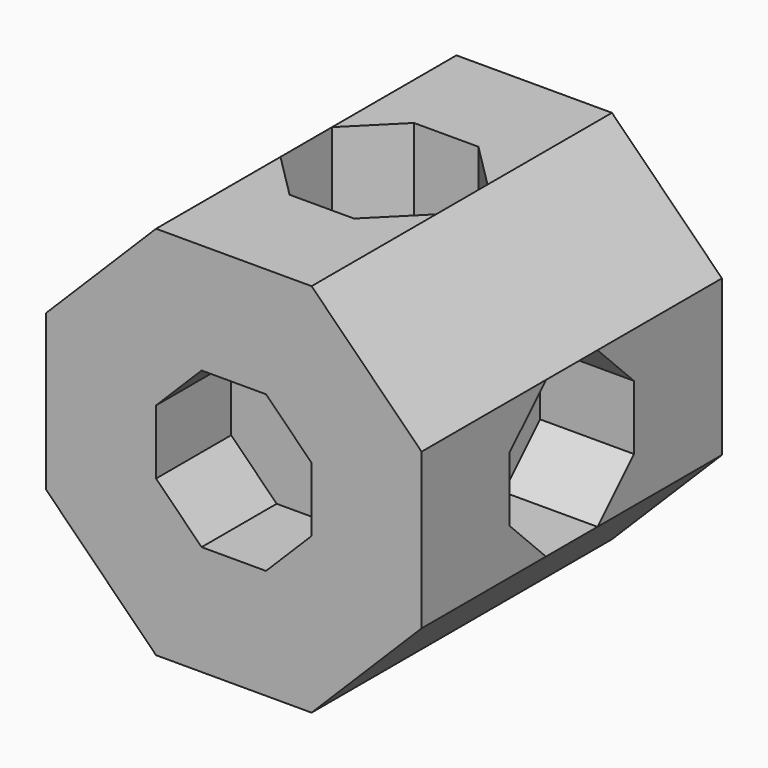
from build123d import *

# Parameters (mm, degrees)
F1_DEPTH        = 15
F2_DEPTH        = 20
F3_DEPTH        = 5
F5_DEPTH        = 5
F5_COPIES_COUNT = 4


# Not quite as in the source:
# - a pattern or mirror of a feature is missing from the dataset's text; its kind, count and spacing are read off the source's solid


with BuildPart() as f1:
    # F0 (on Front) → F1 (new body)
    with BuildSketch(Plane.XZ):
        Polygon((-4.1421356237, -1.7157287525), (-1.7157287525, -4.1421356237), (1.7157287525, -4.1421356237), (4.1421356237, -1.7157287525), (4.1421356237, 1.7157287525), (1.7157287525, 4.1421356237), (-1.7157287525, 4.1421356237), (-4.1421356237, 1.7157287525), align=None)
    extrude(amount=F1_DEPTH)

    # F0 (on Front) → F2 (join)
    with BuildSketch(Plane.XZ):
        Polygon((4.1421356237, -10), (10, -4.1421356237), (10, 4.1421356237), (4.1421356237, 10), (-4.1421356237, 10), (-10, 4.1421356237), (-10, -4.1421356237), (-4.1421356237, -10), align=None)
        Polygon((1.7157287525, -4.1421356237), (-1.7157287525, -4.1421356237), (-4.1421356237, -1.7157287525), (-4.1421356237, 1.7157287525), (-1.7157287525, 4.1421356237), (1.7157287525, 4.1421356237), (4.1421356237, 1.7157287525), (4.1421356237, -1.7157287525), align=None, mode=Mode.SUBTRACT)
    extrude(amount=F2_DEPTH)

    # F0 (on Front) → F3 (cut)
    with BuildSketch(Plane.XZ):
        Polygon((-4.1421356237, -1.7157287525), (-1.7157287525, -4.1421356237), (1.7157287525, -4.1421356237), (4.1421356237, -1.7157287525), (4.1421356237, 1.7157287525), (1.7157287525, 4.1421356237), (-1.7157287525, 4.1421356237), (-4.1421356237, 1.7157287525), align=None)
    extrude(amount=F3_DEPTH, mode=Mode.SUBTRACT)

    # F4 (on face) → F5 (cut)
    with BuildSketch(Plane(origin=(0, 0, -10), x_dir=(1, 0, 0), z_dir=(0, 0, -1))):
        Polygon((-4.1421356237, 11.7157287525), (-4.1421356237, 8.2842712475), (-1.7157287525, 5.8578643763), (1.7157287525, 5.8578643763), (4.1421356237, 8.2842712475), (4.1421356237, 11.7157287525), (1.7157287525, 14.1421356237), (-1.7157287525, 14.1421356237), align=None)
    f5 = extrude(amount=-F5_DEPTH, mode=Mode.SUBTRACT)

    # F5_copies: F5 ×4 about axis
    f5_copies_axis = Axis((0, 0, 0), (0, 1, 0))
    for i in range(1, F5_COPIES_COUNT):
        add(f5.rotate(f5_copies_axis, i * 360 / F5_COPIES_COUNT), mode=Mode.SUBTRACT)


solid = f1.part
